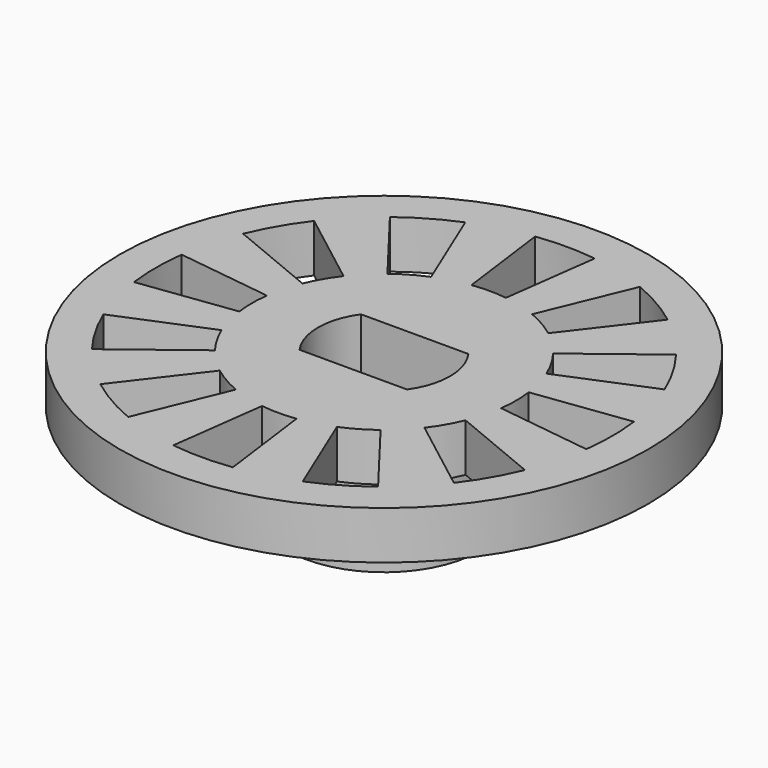
from build123d import *

# Parameters (mm, degrees)
F0_R            = 11
F1_DEPTH        = 2
F3_DEPTH        = 2
F3_COPIES_COUNT = 12
F4_R            = 4
F5_DEPTH        = 4
F7_DEPTH        = 9


# Not quite as in the source:
# - a pattern or mirror of a feature is missing from the dataset's text; its kind, count and spacing are read off the source's solid


with BuildPart() as f1:
    # F0 (on Top) → F1 (new body)
    with BuildSketch(Plane.XY):
        Circle(F0_R)
    extrude(amount=F1_DEPTH)

    # F2 (on face) → F3 (cut)
    with BuildSketch(Plane.XY.offset(2)):
        with BuildLine():
            Line((9.4187261831, 1.2399988261), (5.4529467376, 0.7178940572))
            ThreePointArc((5.4529467376, 0.7178940572), (5.5, 0), (5.4529467376, -0.7178940572))
            Line((5.4529467376, -0.7178940572), (9.4187261831, -1.2399988261))
            ThreePointArc((9.4187261831, -1.2399988261), (9.5, 0), (9.4187261831, 1.2399988261))
        make_face()
    f3 = extrude(amount=-F3_DEPTH, mode=Mode.SUBTRACT)

    # F3_copies: F3 ×12 about axis
    f3_copies_axis = Axis((0, 0, 0), (0, 0, 1))
    for i in range(1, F3_COPIES_COUNT):
        add(f3.rotate(f3_copies_axis, i * 360 / F3_COPIES_COUNT), mode=Mode.SUBTRACT)

    # F4 (on face) → F5 (join)
    with BuildSketch(Plane(origin=(0, 0, 0), x_dir=(1, 0, 0), z_dir=(0, 0, -1))):
        Circle(F4_R)
    extrude(amount=F5_DEPTH)

    # F6 (on face) → F7 (cut)
    with BuildSketch(Plane(origin=(0, 0, -4), x_dir=(1, 0, 0), z_dir=(0, 0, -1))):
        with BuildLine():
            Line((-2.2366269246, -1.6), (2.2366269246, -1.6))
            ThreePointArc((2.2366269246, -1.6), (2.75, 0), (2.2366269246, 1.6))
            Line((2.2366269246, 1.6), (-2.2366269246, 1.6))
            ThreePointArc((-2.2366269246, 1.6), (-2.75, 0), (-2.2366269246, -1.6))
        make_face()
    extrude(amount=-F7_DEPTH, mode=Mode.SUBTRACT)


solid = f1.part
